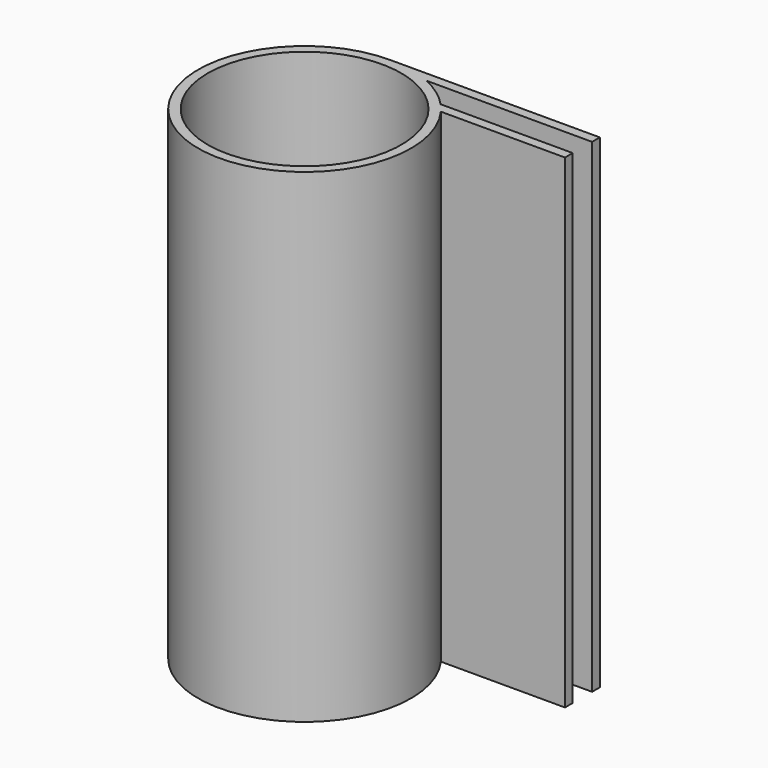
from build123d import *

# Parameters (mm, degrees)
F0_R     = 10
F1_DEPTH = 50
F2_D     = 20
F2_DEPTH = 51
F2_TIP   = 6.0086061903


# Not quite as in the source:
# - a feature names something its author has since deleted; it is built from what else it names


with BuildPart() as f1:
    # F0 (on Top) → F1 (new body)
    with BuildSketch(Plane.XY):
        with BuildLine():
            Line((0, 19.2077464238), (-13.6434029399, 19.2077464238))
            ThreePointArc((-13.6434029399, 19.2077464238), (-15.252953043, 20.6275337493), (-17.1075657147, 21.7077464238))
            Line((-17.1075657147, 21.7077464238), (0, 21.7077464238))
            Line((0, 21.7077464238), (0, 22.7077464238))
            Line((0, 22.7077464238), (-21.6901414096, 22.7077464238))
            ThreePointArc((-21.6901414096, 22.7077464238), (-26.6650785952, 1.8970379886), (-12.816021735, 18.2077464238))
            Line((-12.816021735, 18.2077464238), (0, 18.2077464238))
            Line((0, 18.2077464238), (0, 19.2077464238))
        make_face()
        with Locations((-21.6901414096, 11.7077464238)):
            Circle(F0_R, mode=Mode.SUBTRACT)
        with Locations((-21.6901414096, 11.7077464238)):
            Circle(F0_R)
    extrude(amount=F1_DEPTH)

    # F2
    with Locations(Plane(origin=(0, 0, 0), x_dir=(1, 0, 0), z_dir=(0, 0, -1))):
        with Locations((-21.6901414096, -11.7077464238)):
            Hole(F2_D / 2, depth=F2_DEPTH)
            with Locations((0, 0, -(F2_DEPTH + F2_TIP / 2))):  # 118° drill point
                Cone(0, F2_D / 2, F2_TIP, mode=Mode.SUBTRACT)


solid = f1.part
